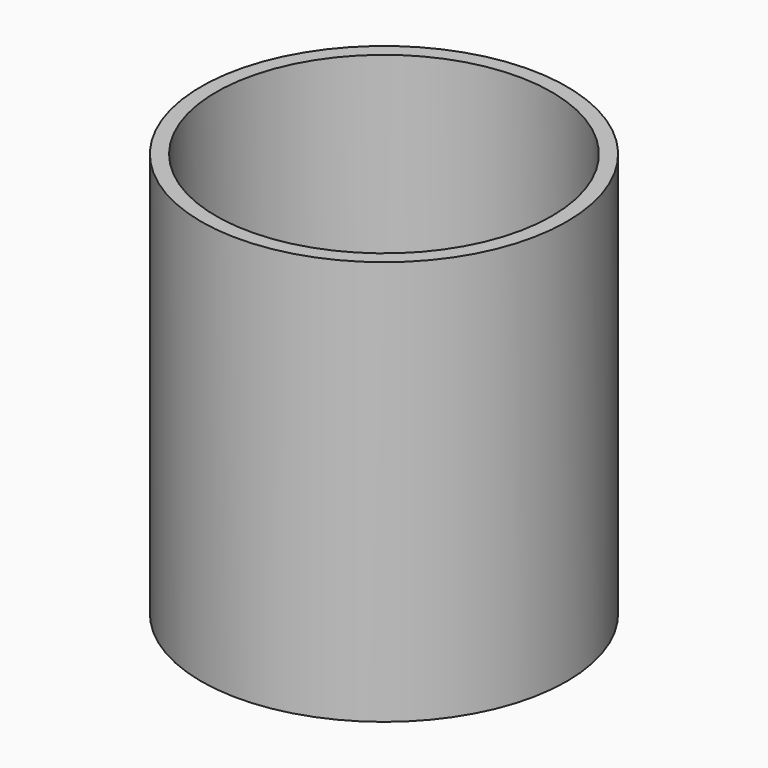
from build123d import *

# Parameters (mm, degrees)
F2_R         = 12.2
F3_DEPTH     = 27
F4_R         = 11.2
F5_DEPTH     = 25
F6_TEXT_SIZE = 6.9444444444
F7_DEPTH     = 1


# Not quite as in the source:
# - Text() gives the source's letters only with a copy of the font that has no kerning and outlines rounded to 1/6400 em; it was checked with that copy


with BuildPart() as f3:
    # F2 (on Top) → F3 (new body)
    with BuildSketch(Plane.XY):
        Circle(F2_R)
    extrude(amount=F3_DEPTH)

    # F4 (on face) → F5 (cut)
    with BuildSketch(Plane.XY.offset(27)):
        Circle(F4_R)
    extrude(amount=-F5_DEPTH, mode=Mode.SUBTRACT)

    # F6 (on face) → F7 (join)
    with BuildSketch(Plane.XY.offset(2)):
        with Locations((-5.9467230903, -2.5)):
            Text('3E8', F6_TEXT_SIZE, font='Open Sans', text_align=(TextAlign.LEFT, TextAlign.BOTTOM))
    extrude(amount=F7_DEPTH)


solid = f3.part
